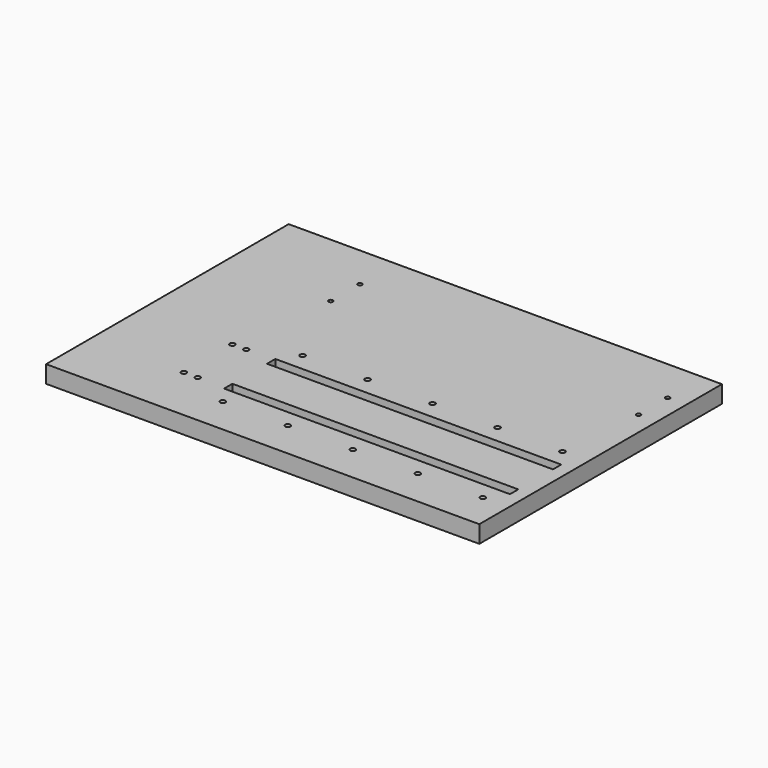
from build123d import *

# Parameters (mm, degrees)
F0_W     = 500
F0_H     = 350
F0_R     = 3
F0_R_2   = 2.5
F0_W_2   = 330
F0_H_2   = 12
F1_DEPTH = 20
F2_DEPTH = 9
F3_DEPTH = 20


# Not quite as in the source:
# - a feature names something its author has since deleted; it is built from what else it names


with BuildPart() as f1:
    # F0 (on Top) → F1 (new body)
    with BuildSketch(Plane.XY):
        with Locations((250, 175)):
            Rectangle(F0_W, F0_H)
        with Locations((107, 65)):
            Circle(F0_R, mode=Mode.SUBTRACT)
        with Locations((123, 65)):
            Circle(F0_R, mode=Mode.SUBTRACT)
        with Locations((107, 135)):
            Circle(F0_R, mode=Mode.SUBTRACT)
        with Locations((123, 135)):
            Circle(F0_R, mode=Mode.SUBTRACT)
        with Locations((170, 42.5)):
            Circle(F0_R, mode=Mode.SUBTRACT)
        with Locations((245, 42.5)):
            Circle(F0_R, mode=Mode.SUBTRACT)
        with Locations((123.3851659298, 256.5)):
            Circle(F0_R_2, mode=Mode.SUBTRACT)
        with Locations((123.4573769569, 298.5)):
            Circle(F0_R_2, mode=Mode.SUBTRACT)
        with Locations((170, 157.5)):
            Circle(F0_R, mode=Mode.SUBTRACT)
        with Locations((245, 157.5)):
            Circle(F0_R, mode=Mode.SUBTRACT)
        with Locations((320, 42.5)):
            Circle(F0_R, mode=Mode.SUBTRACT)
        with Locations((320, 69)):
            Rectangle(F0_W_2, F0_H_2, mode=Mode.SUBTRACT)
        with Locations((320, 131)):
            Rectangle(F0_W_2, F0_H_2, mode=Mode.SUBTRACT)
        with Locations((395, 42.5)):
            Circle(F0_R, mode=Mode.SUBTRACT)
        with Locations((470, 42.5)):
            Circle(F0_R, mode=Mode.SUBTRACT)
        with Locations((320, 157.5)):
            Circle(F0_R, mode=Mode.SUBTRACT)
        with Locations((395, 157.5)):
            Circle(F0_R, mode=Mode.SUBTRACT)
        with Locations((470, 157.5)):
            Circle(F0_R, mode=Mode.SUBTRACT)
        with Locations((478.6148340702, 256.5)):
            Circle(F0_R_2, mode=Mode.SUBTRACT)
        with Locations((478.5426230431, 298.5)):
            Circle(F0_R_2, mode=Mode.SUBTRACT)
        with Locations((320, 131)):
            Rectangle(F0_W_2, F0_H_2)
        with Locations((245, 157.5)):
            Circle(F0_R)
        with Locations((395, 157.5)):
            Circle(F0_R)
        with Locations((470, 42.5)):
            Circle(F0_R)
        with Locations((395, 42.5)):
            Circle(F0_R)
        with Locations((320, 42.5)):
            Circle(F0_R)
        with Locations((170, 42.5)):
            Circle(F0_R)
        with Locations((245, 42.5)):
            Circle(F0_R)
        with Locations((123, 65)):
            Circle(F0_R)
        with Locations((107, 65)):
            Circle(F0_R)
        with Locations((123, 135)):
            Circle(F0_R)
        with Locations((170, 157.5)):
            Circle(F0_R)
        with Locations((320, 157.5)):
            Circle(F0_R)
        with Locations((470, 157.5)):
            Circle(F0_R)
        with Locations((107, 135)):
            Circle(F0_R)
        with Locations((478.5426230431, 298.5)):
            Circle(F0_R_2)
        with Locations((478.6148340702, 256.5)):
            Circle(F0_R_2)
        with Locations((123.4573769569, 298.5)):
            Circle(F0_R_2)
        with Locations((123.3851659298, 256.5)):
            Circle(F0_R_2)
        with Locations((320, 69)):
            Rectangle(F0_W_2, F0_H_2)
    extrude(amount=-F1_DEPTH)

    # F0 (on Top) → F2 (cut)
    with BuildSketch(Plane.XY):
        with Locations((320, 131)):
            Rectangle(F0_W_2, F0_H_2)
        with Locations((320, 69)):
            Rectangle(F0_W_2, F0_H_2)
    extrude(amount=-F2_DEPTH, mode=Mode.SUBTRACT)

    # F0 (on Top) → F3 (cut)
    with BuildSketch(Plane.XY):
        with Locations((170, 42.5)):
            Circle(F0_R)
        with Locations((245, 42.5)):
            Circle(F0_R)
        with Locations((320, 42.5)):
            Circle(F0_R)
        with Locations((395, 42.5)):
            Circle(F0_R)
        with Locations((470, 42.5)):
            Circle(F0_R)
        with Locations((470, 157.5)):
            Circle(F0_R)
        with Locations((395, 157.5)):
            Circle(F0_R)
        with Locations((320, 157.5)):
            Circle(F0_R)
        with Locations((245, 157.5)):
            Circle(F0_R)
        with Locations((170, 157.5)):
            Circle(F0_R)
        with Locations((107, 135)):
            Circle(F0_R)
        with Locations((123, 135)):
            Circle(F0_R)
        with Locations((123, 65)):
            Circle(F0_R)
        with Locations((107, 65)):
            Circle(F0_R)
        with Locations((478.5426230431, 298.5)):
            Circle(F0_R_2)
        with Locations((478.6148340702, 256.5)):
            Circle(F0_R_2)
        with Locations((123.3851659298, 256.5)):
            Circle(F0_R_2)
        with Locations((123.4573769569, 298.5)):
            Circle(F0_R_2)
    extrude(amount=-F3_DEPTH, mode=Mode.SUBTRACT)


solid = f1.part
